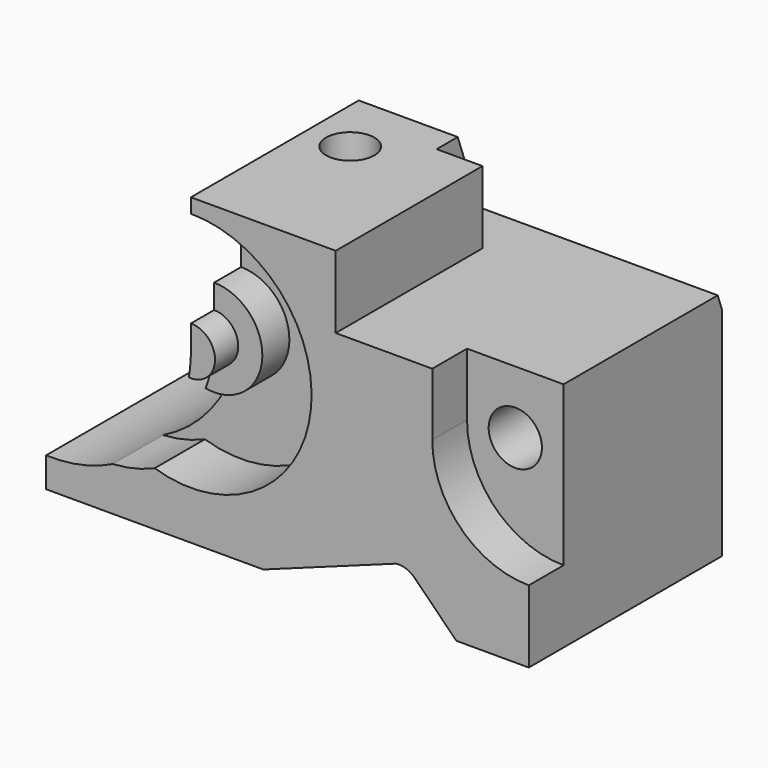
from build123d import *

# Parameters (mm, degrees)
F0_R      = 5.5120501068
F1_DEPTH  = 50
F3_DEPTH  = 13
F4_R      = 10
F5_DEPTH  = 7
F6_R      = 5
F7_DEPTH  = 6
F8_R      = 5.5120501068
F9_DEPTH  = 9
F11_DEPTH = 381
F13_DEPTH = 381
F14_W     = 50
F14_H     = 12
F15_DEPTH = 15
F16_R     = 5
F17_DEPTH = 381


with BuildPart() as f1:
    # F0 (on Front) → F1 (new body)
    with BuildSketch(Plane.XZ):
        with BuildLine():
            Line((60, -15), (60, 0))
            Line((60, 0), (0, 0))
            Line((0, 0), (0, -63))
            Line((0, -63), (45, -63))
            Line((45, -63), (72.4561188247, -53.0067899993))
            ThreePointArc((72.4561188247, -53.0067899993), (74.5109412295, -53.1845320084), (76.2667195414, -54.2667195414))
            Line((76.2667195414, -54.2667195414), (85, -63))
            Line((85, -63), (100, -63))
            Line((100, -63), (100, -15))
            Line((100, -15), (60, -15))
        make_face()
        with Locations((90, -28)):
            Circle(F0_R, mode=Mode.SUBTRACT)
    extrude(amount=F1_DEPTH)

    # F2 (on face) → F3 (cut)
    with BuildSketch(Plane.XZ.offset(50)):
        with BuildLine():
            Line((30, 0), (0, 0))
            Line((0, 0), (0, -50.6242252886))
            ThreePointArc((0, -50.6242252886), (11.1042474662, -53.9150696691), (22.5, -51.8484800354))
            ThreePointArc((22.5, -51.8484800354), (54.7104431454, -31.7939424821), (30, -3))
            Line((30, -3), (30, 0))
        make_face()
    extrude(amount=-F3_DEPTH, mode=Mode.SUBTRACT)

    # F4 (on face) → F5 (join)
    with BuildSketch(Plane.XZ.offset(37)):
        with Locations((30, -28)):
            Circle(F4_R)
    extrude(amount=F5_DEPTH)

    # F6 (on face) → F7 (join)
    with BuildSketch(Plane.XZ.offset(44)):
        with Locations((30, -28)):
            Circle(F6_R)
    extrude(amount=F7_DEPTH)

    # F8 (on face) → F9 (cut)
    with BuildSketch(Plane.XZ.offset(50)):
        with BuildLine():
            Line((100, -15), (80, -15))
            Line((80, -15), (80, -28))
            ThreePointArc((80, -28), (85.8578643763, -42.1421356237), (100, -48))
            Line((100, -48), (100, -15))
        make_face()
        with Locations((90, -28)):
            Circle(F8_R, mode=Mode.SUBTRACT)
    extrude(amount=-F9_DEPTH, mode=Mode.SUBTRACT)

    # F10 (on face) → F11 (cut)
    with BuildSketch(Plane.XZ.offset(50)):
        with BuildLine():
            Line((30, 0), (0, 0))
            Line((0, 0), (0, -56.8121126443))
            ThreePointArc((0, -56.8121126443), (21.1383307761, -48.7974627961), (30, -28))
            Line((30, -28), (30, 0))
        make_face()
    extrude(amount=-F11_DEPTH, mode=Mode.SUBTRACT)

    # F12 (on face) → F13 (cut)
    with BuildSketch(Plane(origin=(30, 0, 0), x_dir=(0, -1, 0), z_dir=(-1, 0, 0))):
        Polygon((6.5514642168, 0), (0, 0), (0, -18), align=None)
    extrude(amount=-F13_DEPTH, mode=Mode.SUBTRACT)

    # F14 (on Top) → F15 (cut)
    with BuildSketch(Plane.XY):
        with Locations((75.5128398538, -6)):
            Rectangle(F14_W, F14_H)
    extrude(amount=-F15_DEPTH, mode=Mode.SUBTRACT)

    # F16 (on face) → F17 (cut)
    with BuildSketch(Plane.XY):
        with Locations((39, -20)):
            Circle(F16_R)
    extrude(amount=-F17_DEPTH, mode=Mode.SUBTRACT)


solid = f1.part
